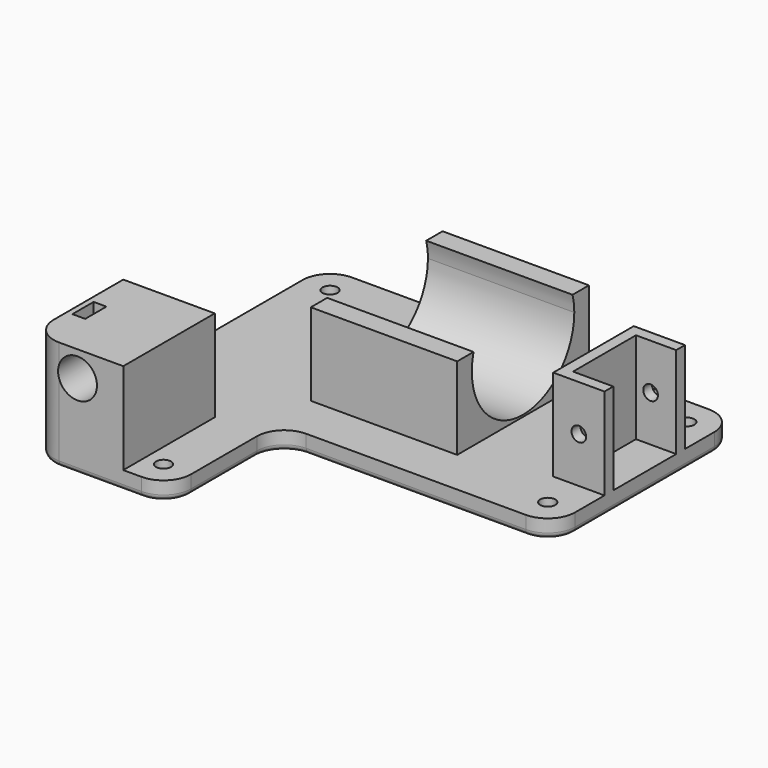
from build123d import *

# Parameters (mm, degrees)
F1_DEPTH        = 4
F2_W            = 32
F2_H            = 36
F3_DEPTH        = 18
F5_DEPTH        = 32
F2_W_2          = 20
F2_H_2          = 25
F6_DEPTH        = 20
F7_R            = 4.25
F8_DEPTH        = 25
F9_W            = 2.8
F9_H            = 5.8
F10_DEPTH       = 12
F11_R           = 1.6
F12_DEPTH       = 10
F13_T1_DEPTH    = 4
F13_T3_DEPTH    = 34
F13_T5_DEPTH    = 54
F2_W_3          = 8.8
F2_H_3          = 2.4
F14_DEPTH       = 20
F15_R           = 1.6
F16_DEPTH       = 22
F18_D           = 3.3
F18_CSINK_D     = 6.72
F18_CSINK_ANGLE = 90
F19_R           = 1.2


# Not quite as in the source:
# - a fillet or chamfer that OpenCascade refuses, or shapes differently, is made with other operations: its cross-section is extruded or revolved along the edge and cut away or added


with BuildPart() as f1:
    # F0 (on Top) → F1 (new body)
    with BuildSketch(Plane.XY):
        Polygon((-45, -40), (-15, -40), (-15, -10), (45, -10), (45, 40), (-45, 40), align=None)
    extrude(amount=F1_DEPTH)

    # F2 (on face) → F3 (join)
    with BuildSketch(Plane.XY.offset(4)):
        with Locations((0, 18)):
            Rectangle(F2_W, F2_H)
    extrude(amount=F3_DEPTH)

    # F4 (on face) → F5 (cut, through all)
    with BuildSketch(Plane.YZ.offset(16)):
        with BuildLine():
            ThreePointArc((4.4707723798, 22), (16.1846745035, 4.5181920003), (32, 18.4))
            ThreePointArc((32, 18.4), (31.8818079997, 20.2153254965), (31.5292276202, 22))
            Line((31.5292276202, 22), (4.4707723798, 22))
        make_face()
    extrude(amount=-F5_DEPTH, mode=Mode.SUBTRACT)

    # F2 (on face) → F6 (join)
    with BuildSketch(Plane.XY.offset(4)):
        with Locations((-35, -27.5)):
            Rectangle(F2_W_2, F2_H_2)
    extrude(amount=F6_DEPTH)

    # F7 (on face) → F8 (cut, through all)
    with BuildSketch(Plane.XZ.offset(40)):
        with Locations((-35, 18.4)):
            Circle(F7_R)
    extrude(amount=-F8_DEPTH, mode=Mode.SUBTRACT)

    # F9 (on face) → F10 (cut)
    with BuildSketch(Plane.XY.offset(24)):
        with Locations((-42.4, -27.5)):
            Rectangle(F9_W, F9_H)
    extrude(amount=-F10_DEPTH, mode=Mode.SUBTRACT)

    # F11 (on face) → F12 (cut)
    with BuildSketch(Plane(origin=(-45, 0, 0), x_dir=(0, -1, 0), z_dir=(-1, 0, 0))):
        with Locations((27.5, 18.4)):
            Circle(F11_R)
    extrude(amount=-F12_DEPTH, mode=Mode.SUBTRACT)

    # F13: fillet of radius 6 on 6 edges, made by hand

    # F13_s2 → F13_t1 (join)
    with BuildSketch(Plane.XY):
        with BuildLine():
            ThreePointArc((-15, -16), (-13.2426406871, -11.7573593129), (-9, -10))
            Line((-9, -10), (-15, -10))
            Line((-15, -10), (-15, -16))
        make_face()
    extrude(amount=F13_T1_DEPTH)

    # F13_s4 → F13_t3 (cut)
    with BuildSketch(Plane.XY.offset(-15)):
        with BuildLine():
            ThreePointArc((-21, -40), (-16.7573593129, -38.2426406871), (-15, -34))
            Line((-15, -34), (-15, -40))
            Line((-15, -40), (-21, -40))
        make_face()
        with BuildLine():
            ThreePointArc((39, -10), (43.2426406871, -8.2426406871), (45, -4))
            Line((45, -4), (45, -10))
            Line((45, -10), (39, -10))
        make_face()
        with BuildLine():
            ThreePointArc((39, 40), (43.2426406871, 38.2426406871), (45, 34))
            Line((45, 34), (45, 40))
            Line((45, 40), (39, 40))
        make_face()
        with BuildLine():
            ThreePointArc((-45, 34), (-43.2426406871, 38.2426406871), (-39, 40))
            Line((-39, 40), (-45, 40))
            Line((-45, 40), (-45, 34))
        make_face()
    extrude(amount=F13_T3_DEPTH, mode=Mode.SUBTRACT)

    # F13_s6 → F13_t5 (cut)
    with BuildSketch(Plane.XY.offset(-15)):
        with BuildLine():
            ThreePointArc((-39, -40), (-43.2426406871, -38.2426406871), (-45, -34))
            Line((-45, -34), (-45, -40))
            Line((-45, -40), (-39, -40))
        make_face()
    extrude(amount=F13_T5_DEPTH, mode=Mode.SUBTRACT)

    # F2 (on face) → F14 (join)
    with BuildSketch(Plane.XY.offset(4)):
        Polygon((36.2, 23.6), (36.2, 26), (33.8, 26), (33.8, 4), (36.2, 4), (36.2, 6.4), align=None)
        with Locations((40.6, 5.2)):
            Rectangle(F2_W_3, F2_H_3)
        with Locations((40.6, 24.8)):
            Rectangle(F2_W_3, F2_H_3)
    extrude(amount=F14_DEPTH)

    # F15 (on face) → F16 (cut, through all)
    with BuildSketch(Plane.XZ.offset(-4)):
        with Locations((39.4, 14)):
            Circle(F15_R)
    extrude(amount=-F16_DEPTH, mode=Mode.SUBTRACT)

    # F18 (through all)
    with Locations(Plane(origin=(0, 0, 0), x_dir=(1, 0, 0), z_dir=(0, 0, -1))):
        with Locations((-21, 34), (39, 4), (39, -34), (-39, -34)):
            CounterSinkHole(F18_D / 2, F18_CSINK_D / 2, counter_sink_angle=F18_CSINK_ANGLE)

    # F19
    f19_edges = [f1.edges().sort_by_distance(p)[0] for p in [
        (0, 40, 0),
        (-43.242641, 38.242641, 0),
        (-30, -40, 0),
        (-43.242641, -38.242641, 0),
        (-45, 0, 0),
        (43.242641, 38.242641, 0),
        (45, 15, 0),
        (-16.757359, -38.242641, 0),
        (43.242641, -8.242641, 0),
        (-15, -25, 0),
        (15, -10, 0),
        (-13.242641, -11.757359, 0),
    ]]
    fillet(f19_edges, radius=F19_R)


solid = f1.part
